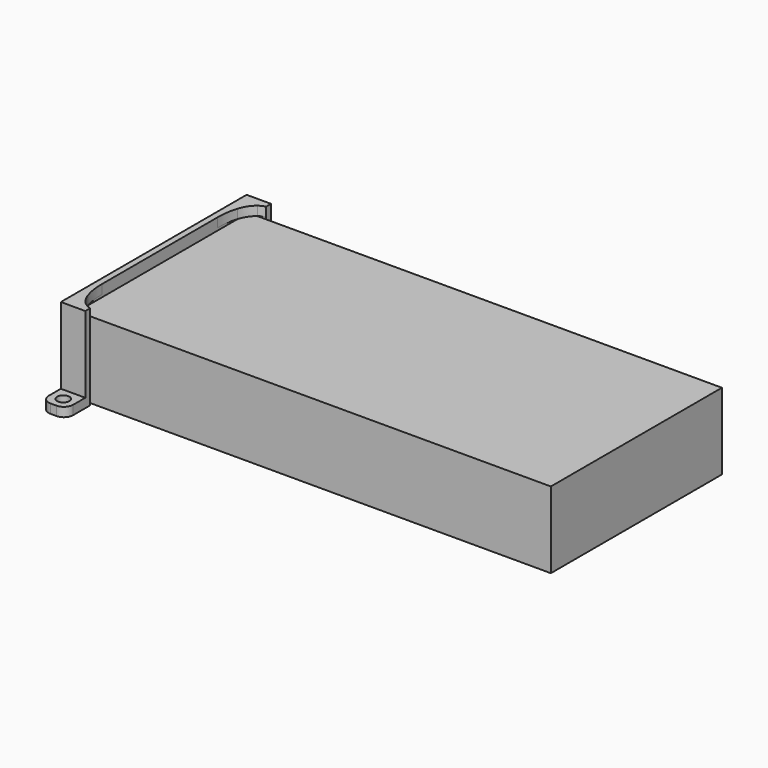
from build123d import *

# Parameters (mm, degrees)
F0_W     = 155
F0_H     = 70
F1_DEPTH = 25
F2_R     = 2
F3_DEPTH = 3
F4_DEPTH = 28
F5_START = 25
F5_DEPTH = 3
F7_DEPTH = 25


# Not quite as in the source:
# - a feature names something its author has since deleted; it is built from what else it names


with BuildPart() as f1:
    # F0 (on Top) → F1 (new body)
    with BuildSketch(Plane.XY):
        with Locations((8.0986786634, -14.300759537)):
            Rectangle(F0_W, F0_H)
    extrude(amount=F1_DEPTH)


with BuildPart() as f3:
    # F2 (on Top) → F3 (new body)
    with BuildSketch(Plane.XY):
        with BuildLine():
            Line((-72.4013213366, 23.699240463), (-64.4013213366, 23.699240463))
            Line((-64.4013213366, 23.699240463), (-64.4013213366, 28.699240463))
            ThreePointArc((-64.4013213366, 28.699240463), (-65.2800009931, 30.8205608065), (-67.4013213366, 31.699240463))
            Line((-67.4013213366, 31.699240463), (-69.4013213366, 31.699240463))
            ThreePointArc((-69.4013213366, 31.699240463), (-71.5226416802, 30.8205608065), (-72.4013213366, 28.699240463))
            Line((-72.4013213366, 28.699240463), (-72.4013213366, 23.699240463))
        make_face()
        with Locations((-68.4013213366, 27.699240463)):
            Circle(F2_R, mode=Mode.SUBTRACT)
        Polygon((-70.4013213366, -14.300759537), (-70.4013213366, 9.3950822393), (-70.4013213366, 21.699240463), (-64.4013213366, 21.699240463), (-64.4013213366, 23.699240463), (-72.4013213366, 23.699240463), (-72.4013213366, -14.300759537), align=None)
        Polygon((-70.4013213366, -50.300759537), (-70.4013213366, -37.9966013134), (-70.4013213366, -14.300759537), (-72.4013213366, -14.300759537), (-72.4013213366, -52.300759537), (-64.4013213366, -52.300759537), (-64.4013213366, -50.300759537), align=None)
        with BuildLine():
            Line((-64.4013213366, -57.300759537), (-64.4013213366, -52.300759537))
            Line((-64.4013213366, -52.300759537), (-72.4013213366, -52.300759537))
            Line((-72.4013213366, -52.300759537), (-72.4013213366, -57.300759537))
            ThreePointArc((-72.4013213366, -57.300759537), (-71.5226416802, -59.4220798806), (-69.4013213366, -60.300759537))
            Line((-69.4013213366, -60.300759537), (-67.4013213366, -60.300759537))
            ThreePointArc((-67.4013213366, -60.300759537), (-65.2800009931, -59.4220798806), (-64.4013213366, -57.300759537))
        make_face()
        with Locations((-68.4013213366, -56.300759537)):
            Circle(F2_R, mode=Mode.SUBTRACT)
    extrude(amount=F3_DEPTH)

    # F2 (on Top) → F4 (join, through all)
    with BuildSketch(Plane.XY):
        Polygon((-70.4013213366, -50.300759537), (-70.4013213366, -37.9966013134), (-70.4013213366, -14.300759537), (-72.4013213366, -14.300759537), (-72.4013213366, -52.300759537), (-64.4013213366, -52.300759537), (-64.4013213366, -50.300759537), align=None)
        Polygon((-70.4013213366, -14.300759537), (-70.4013213366, 9.3950822393), (-70.4013213366, 21.699240463), (-64.4013213366, 21.699240463), (-64.4013213366, 23.699240463), (-72.4013213366, 23.699240463), (-72.4013213366, -14.300759537), align=None)
    extrude(amount=F4_DEPTH)

    # F2 (on Top) → F5 (join)
    with BuildSketch(Plane.XY.offset(F5_START)):
        with BuildLine():
            Line((-66.5030320211, 20.699240463), (-69.4013213366, 20.699240463))
            Line((-69.4013213366, 20.699240463), (-69.4013213366, 16.260107167))
            add(Edge.make_bspline(
                [(-66.5030320211, 20.699240463), (-67.8075846929, 19.7092528514), (-68.7629395105, 18.1494653893), (-69.4013213366, 16.260107167)],
                knots=[2.5629502301, 2.5629502301, 2.5629502301, 2.5629502301, 7.9519487063, 7.9519487063, 7.9519487063, 7.9519487063], degree=3))
        make_face()
        with BuildLine():
            Line((-69.4013213366, 16.260107167), (-69.4013213366, 20.699240463))
            Line((-69.4013213366, 20.699240463), (-66.5030320211, 20.699240463))
            add(Edge.make_bspline(
                [(-64.4013213366, 21.699240463), (-65.1831859383, 21.5120152683), (-65.8826006765, 21.1700680181), (-66.5030320211, 20.699240463)],
                knots=[0, 0, 0, 0, 2.5629502301, 2.5629502301, 2.5629502301, 2.5629502301], degree=3))
            Line((-64.4013213366, 21.699240463), (-70.4013213366, 21.699240463))
            Line((-70.4013213366, 21.699240463), (-70.4013213366, 9.3950822393))
            add(Edge.make_bspline(
                [(-69.4013213366, 16.260107167), (-70.0809490956, 14.2486772642), (-70.4013213366, 11.8637135989), (-70.4013213366, 9.3950822393)],
                knots=[7.9519487063, 7.9519487063, 7.9519487063, 7.9519487063, 13.6891310752, 13.6891310752, 13.6891310752, 13.6891310752], degree=3))
        make_face()
        with BuildLine():
            add(Edge.make_bspline(
                [(-66.5030320211, -49.300759537), (-67.8075846929, -48.3107719254), (-68.7629395105, -46.7509844633), (-69.4013213366, -44.861626241)],
                knots=[2.5629502301, 2.5629502301, 2.5629502301, 2.5629502301, 7.9519487063, 7.9519487063, 7.9519487063, 7.9519487063], degree=3))
            Line((-69.4013213366, -44.861626241), (-69.4013213366, -49.300759537))
            Line((-69.4013213366, -49.300759537), (-66.5030320211, -49.300759537))
        make_face()
        with BuildLine():
            Line((-69.4013213366, -49.300759537), (-69.4013213366, -44.861626241))
            add(Edge.make_bspline(
                [(-69.4013213366, -44.861626241), (-70.0809490956, -42.8501963382), (-70.4013213366, -40.4652326729), (-70.4013213366, -37.9966013134)],
                knots=[7.9519487063, 7.9519487063, 7.9519487063, 7.9519487063, 13.6891310752, 13.6891310752, 13.6891310752, 13.6891310752], degree=3))
            Line((-70.4013213366, -37.9966013134), (-70.4013213366, -50.300759537))
            Line((-70.4013213366, -50.300759537), (-64.4013213366, -50.300759537))
            add(Edge.make_bspline(
                [(-64.4013213366, -50.300759537), (-65.1831859383, -50.1135343424), (-65.8826006765, -49.7715870921), (-66.5030320211, -49.300759537)],
                knots=[0, 0, 0, 0, 2.5629502301, 2.5629502301, 2.5629502301, 2.5629502301], degree=3))
            Line((-66.5030320211, -49.300759537), (-69.4013213366, -49.300759537))
        make_face()
    extrude(amount=F5_DEPTH)

    # F6 (on face) → F7 (cut)
    with BuildSketch(Plane(origin=(-72.4013213366, 0, 0), x_dir=(0, -1, 0), z_dir=(-1, 0, 0))):
        Polygon((-18.09635478, 16.25), (-14.199240463, 14), (-10.302126146, 16.25), (-10.302126146, 20.75), (-14.199240463, 23), (-18.09635478, 20.75), align=None)
        Polygon((-4.199240463, 23), (-8.09635478, 20.75), (-8.09635478, 16.25), (-4.199240463, 14), (-0.302126146, 16.25), (-0.302126146, 20.75), align=None)
        Polygon((5.800759537, 23), (1.90364522, 20.75), (1.90364522, 16.25), (5.800759537, 14), (9.697873854, 16.25), (9.697873854, 20.75), align=None)
        Polygon((15.800759537, 23), (11.90364522, 20.75), (11.90364522, 16.25), (15.800759537, 14), (19.697873854, 16.25), (19.697873854, 20.75), align=None)
        Polygon((25.800759537, 23), (21.90364522, 20.75), (21.90364522, 16.25), (25.800759537, 14), (29.697873854, 16.25), (29.697873854, 20.75), align=None)
        Polygon((35.800759537, 23), (31.90364522, 20.75), (31.90364522, 16.25), (35.800759537, 14), (39.697873854, 16.25), (39.697873854, 20.75), align=None)
        Polygon((37.3003223389, 8.3999978378), (41.197436656, 6.1499978378), (45.094550973, 8.3999978378), (45.094550973, 12.8999978378), (41.197436656, 15.1499978378), (37.3003223389, 12.8999978378), align=None)
        Polygon((27.3003223389, 8.3999978378), (31.197436656, 6.1499978378), (35.094550973, 8.3999978378), (35.094550973, 12.8999978378), (31.197436656, 15.1499978378), (27.3003223389, 12.8999978378), align=None)
        Polygon((17.3003223389, 8.3999978378), (21.197436656, 6.1499978378), (25.094550973, 8.3999978378), (25.094550973, 12.8999978378), (21.197436656, 15.1499978378), (17.3003223389, 12.8999978378), align=None)
        Polygon((7.3003223389, 8.3999978378), (11.197436656, 6.1499978378), (15.094550973, 8.3999978378), (15.094550973, 12.8999978378), (11.197436656, 15.1499978378), (7.3003223389, 12.8999978378), align=None)
        Polygon((-2.6996776611, 8.3999978378), (1.197436656, 6.1499978378), (5.094550973, 8.3999978378), (5.094550973, 12.8999978378), (1.197436656, 15.1499978378), (-2.6996776611, 12.8999978378), align=None)
        Polygon((-8.802563344, 15.1499978378), (-12.6996776611, 12.8999978378), (-12.6996776611, 8.3999978378), (-8.802563344, 6.1499978378), (-4.905449027, 8.3999978378), (-4.905449027, 12.8999978378), align=None)
    extrude(amount=-F7_DEPTH, mode=Mode.SUBTRACT)


solid = Compound([f1.part, f3.part])
